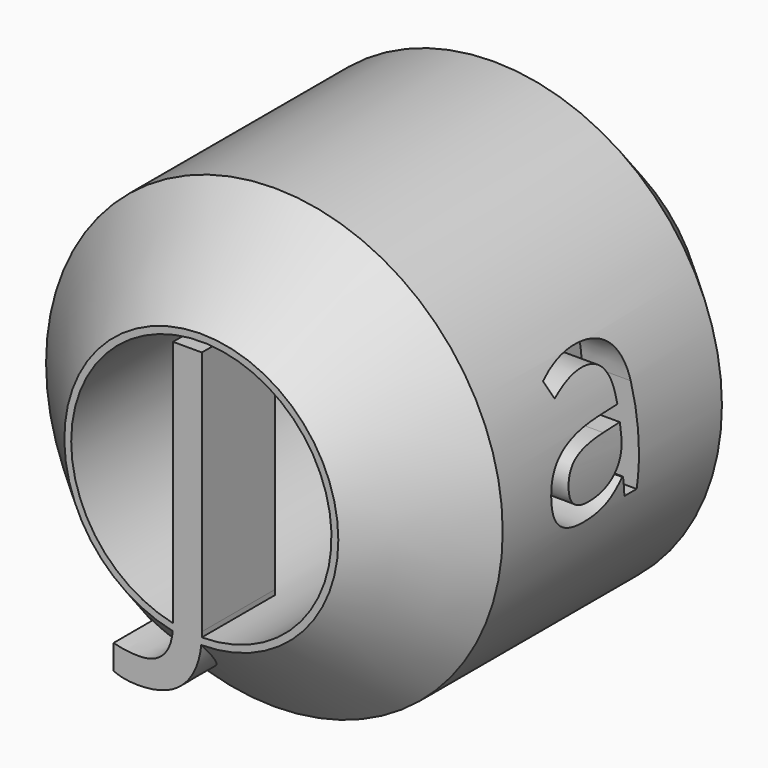
from build123d import *

# Parameters (mm, degrees)
F0_R         = 12.7
F1_DEPTH     = 25.4
F2_SIZE      = 5.08
F3_R         = 7.239
F4_DEPTH     = 25.401
F5_TEXT_SIZE = 14.2039472444
F6_DEPTH     = 5.08
F7_TEXT_SIZE = 19.338172332
F8_DEPTH     = 5.08
F9_TEXT_SIZE = 20.4734064432
F10_DEPTH    = 5.08


# Not quite as in the source:
# - Text() gives the source's letters only with a copy of the font that has no kerning and outlines rounded to 1/6400 em; it was checked with that copy


with BuildPart() as f1:
    # F0 (on Front) → F1 (new body)
    with BuildSketch(Plane.XZ):
        with Locations((-14.5882898942, 27.5222379714)):
            Circle(F0_R)
    extrude(amount=F1_DEPTH)

    # F2
    f2_edges = [f1.edges().sort_by_distance(p)[0] for p in [
        (-27.28829, -25.4, 27.522238),
        (-27.28829, 0, 27.522238),
    ]]
    chamfer(f2_edges, length=F2_SIZE)

    # F3 (on face) → F4 (cut, through all)
    with BuildSketch(Plane(origin=(0, 0, 0), x_dir=(-1, 0, 0), z_dir=(0, 1, 0))):
        with Locations((14.5882898942, 27.5222379714)):
            Circle(F3_R)
    extrude(amount=-F4_DEPTH, mode=Mode.SUBTRACT)

    # F5 (on Right) → F6 (cut)
    with BuildSketch(Plane.YZ):
        with Locations((-17.5961833447, 25.7175005972)):
            Text('a', F5_TEXT_SIZE, font='Open Sans', text_align=(TextAlign.LEFT, TextAlign.BOTTOM))
    extrude(amount=-F6_DEPTH, mode=Mode.SUBTRACT)

    # F7 (on face) → F8 (join)
    with BuildSketch(Plane.XZ.offset(25.4)):
        with Locations((-17.9590255084, 20.4326796616)):
            Text('J', F7_TEXT_SIZE, font='Open Sans', text_align=(TextAlign.LEFT, TextAlign.BOTTOM))
    extrude(amount=-F8_DEPTH)

    # F9 (on face) → F10 (join)
    with BuildSketch(Plane(origin=(0, 0, 0), x_dir=(-1, 0, 0), z_dir=(0, 1, 0))):
        with Locations((9.3411589041, 19.856447354)):
            Text('A', F9_TEXT_SIZE, font='Open Sans', text_align=(TextAlign.LEFT, TextAlign.BOTTOM))
    extrude(amount=-F10_DEPTH)


solid = f1.part
